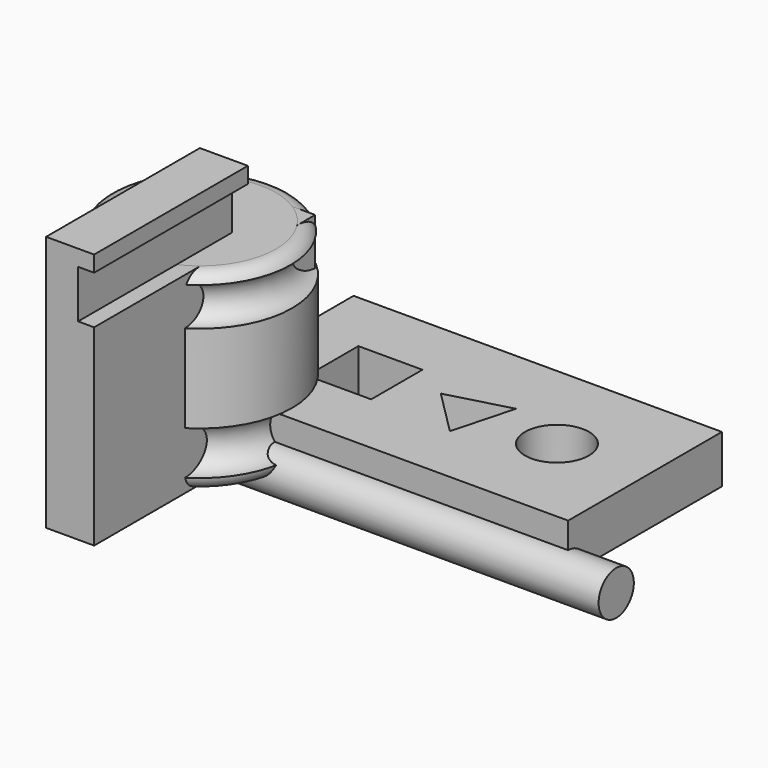
from build123d import *

# Parameters (mm, degrees)
F1_DEPTH  = 76.2
F2_W      = 25.4
F2_H      = 25.4
F3_DEPTH  = 25.4
F4_DEPTH  = 76.2
F6_DEPTH  = 76.2
F7_W      = 146.05
F7_H      = 76.2
F7_W_2    = 25.4
F7_H_2    = 25.4
F7_R      = 12.7
F8_DEPTH  = 19.05
F9_DEPTH  = 19.05
F11_DEPTH = 76.2
F15_D     = 17.4625
F15_DEPTH = 36.5884821235
F16_R     = 8.73125
F17_DEPTH = 165.1


with BuildPart() as f1:
    # F0 (on Top) → F1 (new body)
    with BuildSketch(Plane.XY):
        with BuildLine():
            ThreePointArc((0, -12.7), (8.9802561211, -8.9802561211), (12.7, 0))
            ThreePointArc((12.7, 0), (8.9802561276, 8.9802561145), (1.86e-08, 12.7))
            ThreePointArc((1.86e-08, 12.7), (-8.9802561145, 8.9802561276), (-12.7, 0))
            ThreePointArc((-12.7, 0), (-8.9802561211, -8.9802561211), (0, -12.7))
        make_face()
    extrude(amount=F1_DEPTH)


with BuildPart() as f3:
    # F2 (on Top) → F3 (new body)
    with BuildSketch(Plane.XY):
        with Locations((12.7, 12.7)):
            Rectangle(F2_W, F2_H)
    extrude(amount=F3_DEPTH)

    # F2 (on Top) → F4 (join)
    with BuildSketch(Plane.XY):
        with Locations((12.7, 12.7)):
            Rectangle(F2_W, F2_H)
    extrude(amount=F4_DEPTH)


with BuildPart() as f6:
    # F5 (on Top) → F6 (new body)
    with BuildSketch(Plane.XY):
        Polygon((14.4475684032, -2.5141798996), (-5.0464405389, 13.7690512099), (-9.4011278643, -11.2548713103), align=None)
    extrude(amount=F6_DEPTH)


with BuildPart() as f8:
    # F7 (on Top) → F8 (new body)
    with BuildSketch(Plane.XY):
        with Locations((73.025, 38.1)):
            Rectangle(F7_W, F7_H)
        with Locations((34.925, 38.1)):
            Rectangle(F7_W_2, F7_H_2, mode=Mode.SUBTRACT)
        Polygon((62.03499059, 41.8955028322), (86.5695065778, 48.4695065778), (79.9955028322, 23.93499059), align=None, mode=Mode.SUBTRACT)
        with Locations((111.125, 38.1)):
            Circle(F7_R, mode=Mode.SUBTRACT)
    extrude(amount=F8_DEPTH)

    # F7 (on Top) → F9 (join)
    with BuildSketch(Plane.XY):
        with Locations((73.025, 38.1)):
            Rectangle(F7_W, F7_H)
        with Locations((34.925, 38.1)):
            Rectangle(F7_W_2, F7_H_2, mode=Mode.SUBTRACT)
        Polygon((62.03499059, 41.8955028322), (86.5695065778, 48.4695065778), (79.9955028322, 23.93499059), align=None, mode=Mode.SUBTRACT)
        with Locations((111.125, 38.1)):
            Circle(F7_R, mode=Mode.SUBTRACT)
    extrude(amount=F9_DEPTH)


with BuildPart() as f11:
    # F10 (on Front) → F11 (new body)
    with BuildSketch(Plane.XZ):
        Polygon((0, 101.6), (0, 0), (19.05, 0), (19.05, 76.2), (12.7, 76.2), (12.7, 95.25), (19.05, 95.25), (19.05, 101.6), align=None)
    extrude(amount=F11_DEPTH)


with BuildPart() as f13:
    # F12 (on Front) → F13 (revolve)
    with BuildSketch(Plane.XZ):
        with BuildLine():
            Line((0, 76.2), (0, 0))
            Line((0, 0), (30.2374821235, 0))
            ThreePointArc((30.2374821235, 0), (34.3734750971, 1.5316950986), (36.5141672311, 5.3878544496))
            ThreePointArc((36.5141672311, 5.3878544496), (27.8992712001, 14.1124911453), (36.5874821235, 22.7641216301))
            Line((36.5874821235, 22.7641216301), (36.5874821235, 57.5794217776))
            ThreePointArc((36.5874821235, 57.5794217776), (29.1272723479, 64.7578258969), (36.0132336316, 72.4887865614))
            ThreePointArc((36.0132336316, 72.4887865614), (33.670134548, 75.19222775), (30.2374821235, 76.2))
            Line((30.2374821235, 76.2), (0, 76.2))
        make_face()
    revolve(axis=Axis((0, 0, 38.1), (0, 0, 1)))

    # F15 (through all, one way)
    with BuildSketch(Plane(origin=(0, 0, 0), x_dir=(1, 0, 0), z_dir=(0, 1, 0))):
        with Locations((0, -38.1)):
            Circle(F15_D / 2)
    extrude(amount=-F15_DEPTH, mode=Mode.SUBTRACT)


with BuildPart() as f17:
    # F16 (on Right) → F17 (new body)
    with BuildSketch(Plane.YZ):
        Circle(F16_R)
    extrude(amount=F17_DEPTH)


solid = Compound([f1.part, f3.part, f6.part, f8.part, f11.part, f13.part, f17.part])
